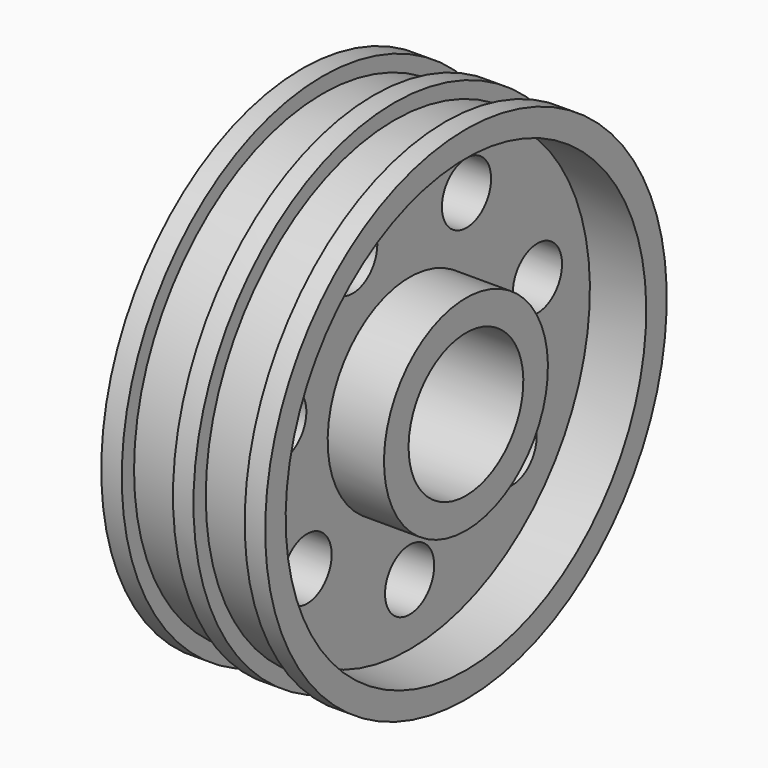
from build123d import *

# Parameters (mm, degrees)
F3_DEPTH        = 533.401
F3_COPIES_COUNT = 7


# Not quite as in the source:
# - a pattern or mirror of a feature is missing from the dataset's text; its kind, count and spacing are read off the source's solid
# - a feature names something its author has since deleted; it is built from what else it names


with BuildPart() as f1:
    # F0 (on Front) → F1 (revolve)
    with BuildSketch(Plane.XZ):
        Polygon((127, 0), (-127, 0), (-127, -609.6), (-406.4, -609.6), (-406.4, -736.6), (-304.8, -736.6), (-304.8, -660.4), (-50.8, -660.4), (-50.8, -736.6), (50.8, -736.6), (50.8, -660.4), (304.8, -660.4), (304.8, -736.6), (406.4, -736.6), (406.4, -609.6), (127, -609.6), align=None)
        Polygon((-406.4, 0), (-127, 0), (127, 0), (406.4, 0), (406.4, 152.4), (0, 152.4), (-406.4, 152.4), align=None)
    revolve(axis=Axis((0, 0, 508), (1, 0, 0)))

    # F2 (on face) → F3 (cut, through all)
    with BuildSketch(Plane(origin=(-127, 0, 0), x_dir=(0, -1, 0), z_dir=(-1, 0, 0))):
        with BuildLine():
            ThreePointArc((152.4, -304.8), (107.7630734528, -197.0369265472), (0, -152.4))
            ThreePointArc((0, -152.4), (-107.7630734528, -412.5630734528), (152.4, -304.8))
        make_face()
    f3 = extrude(amount=-F3_DEPTH, mode=Mode.SUBTRACT)

    # F3_copies: F3 ×7 about axis
    f3_copies_axis = Axis((0, 0, 508), (1, 0, 0))
    for i in range(1, F3_COPIES_COUNT):
        add(f3.rotate(f3_copies_axis, i * 360 / F3_COPIES_COUNT), mode=Mode.SUBTRACT)


solid = f1.part
